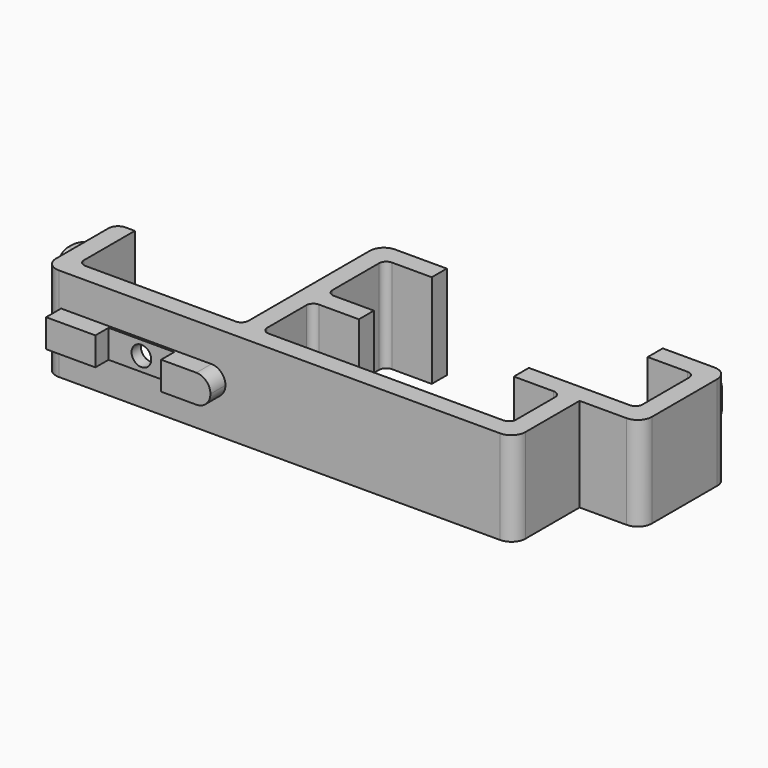
from build123d import *

# Parameters (mm, degrees)
F1_DEPTH = 10
F3_DEPTH = 5
F4_R     = 1.5
F5_R     = 3
F7_DEPTH = 3
F10_R    = 2
F11_R    = 2.99999


# Not quite as in the source:
# - a fillet or chamfer is up to 0.001 mm smaller than in the source, because OpenCascade refuses the exact size


with BuildPart() as f1:
    # F0 (on Top) → F1 (new body, symmetric)
    with BuildSketch(Plane.XY):
        Polygon((0, 0), (-35, 0), (-35, 15), (-39, 15), (-39, -4), (61, -4), (61, 13.4), (74, 13.4), (74, 36.8), (60, 36.8), (60, 32.8), (70, 32.8), (70, 17.4), (47, 17.4), (47, 13.4), (57, 13.4), (57, 0), (4, 0), (4, 13.4), (14, 13.4), (14, 17.4), (4, 17.4), (4, 32.8), (14, 32.8), (14, 36.8), (0, 36.8), align=None)
    extrude(amount=F1_DEPTH, both=True)

    # F2 (on Top) → F3 (join, symmetric)
    with BuildSketch(Plane.XY):
        Polygon((60, 43.8), (60, 36.8), (63, 36.8), (63, 40.8), (67, 40.8), (67, 43.8), align=None)
        Polygon((-43, 12), (-39, 12), (-39, 15), (-46, 15), (-46, 8), (-43, 8), align=None)
    extrude(amount=F3_DEPTH, both=True)

    # F4
    f4_edges = [f1.edges().sort_by_distance(p)[0] for p in [
        (-35, 0, 0),
        (4, 0, 0),
        (4, 17.4, 0),
        (63, 36.8, 0),
        (63, 40.8, 0),
        (4, 32.8, 0),
        (4, 13.4, 0),
        (70, 17.4, 0),
        (57, 0, 0),
        (70, 32.8, 0),
        (57, 13.4, 0),
        (-39, 12, 0),
        (-43, 12, 0),
        (0, 0, 0),
    ]]
    fillet(f4_edges, radius=F4_R)

    # F5
    f5_edges = [f1.edges().sort_by_distance(p)[0] for p in [
        (-39, -4, 0),
        (61, -4, 0),
        (74, 13.4, 0),
        (74, 36.8, 0),
        (60, 43.8, 0),
        (-46, 15, 0),
        (0, 36.8, 0),
        (-44.5, 8, 5),
        (67, 42.3, 5),
        (-44.5, 8, -5),
        (67, 42.3, -5),
    ]]
    fillet(f5_edges, radius=F5_R)

    # F6 (on Top) → F7 (join, symmetric)
    with BuildSketch(Plane.XY):
        Polygon((-11, -8), (-0.5, -8), (-0.5, -4), (-35.5, -4), (-35.5, -8), (-25, -8), (-25, -4.5), (-11, -4.5), align=None)
    extrude(amount=F7_DEPTH, both=True)

    # F8 (on Top) → F9 (revolve, cut)
    with BuildSketch(Plane.XY):
        Polygon((-18, -4.5), (-15.9, -4.5), (-15.9, -2), (-13.75, -2), (-13.75, 0), (-18, 0), align=None)
    revolve(axis=Axis((-18, 1.7481091395, 0), (0, 1, 0)), mode=Mode.SUBTRACT)

    # F10
    f10_edges = [f1.edges().sort_by_distance(p)[0] for p in [
        (-39, 15, -7.5),
        (-39, 15, 7.5),
    ]]
    fillet(f10_edges, radius=F10_R)

    # F11 (radius 3 in the source; OpenCascade refuses exactly that, so slightly less here)
    f11_edges = [f1.edges().sort_by_distance(p)[0] for p in [
        (-0.5, -6, -3),
        (-0.5, -6, 3),
    ]]
    fillet(f11_edges, radius=F11_R)


solid = f1.part
